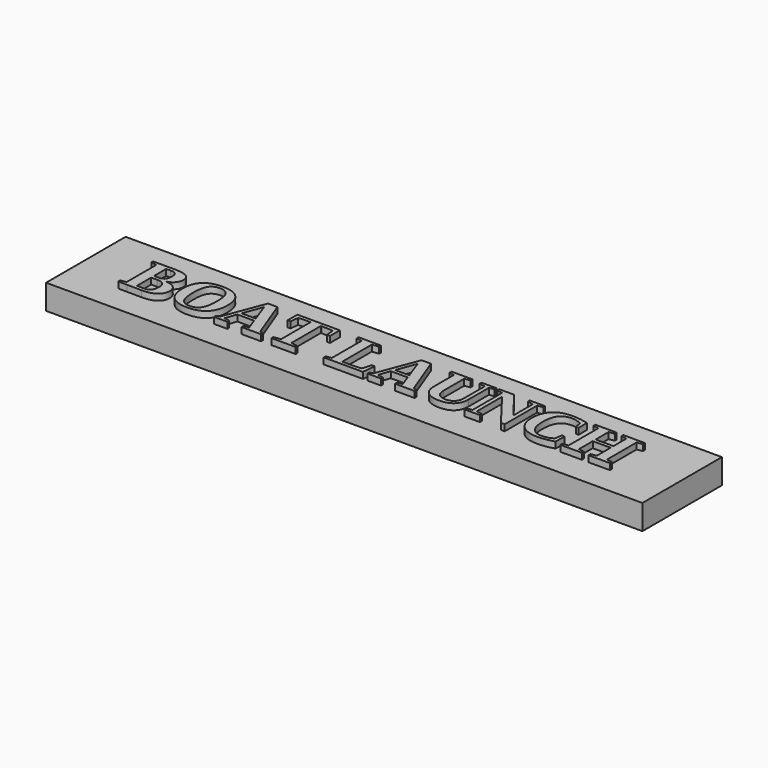
from build123d import *

# Parameters (mm, degrees)
F1_W         = 609.6
F1_H         = 101.6
F2_DEPTH     = 25.4
F0_TEXT_SIZE = 68.0637260033
F3_DEPTH     = 6.35


# Not quite as in the source:
# - Text() gives the source's letters only with a copy of the font that has no kerning and outlines rounded to 1/6400 em; it was checked with that copy


with BuildPart() as f2:
    # F1 (on Top) → F2 (new body)
    with BuildSketch(Plane.XY):
        with Locations((20.5955467701, 29.6312676191)):
            Rectangle(F1_W, F1_H)
    extrude(amount=-F2_DEPTH)

    # F0 (on Top) → F3 (join)
    with BuildSketch(Plane.XY):
        with Locations((-233.9750987422, 6.9081966477)):
            Text('BOAT LAUNCH', F0_TEXT_SIZE, font='Tinos', font_style=FontStyle.BOLD, text_align=(TextAlign.LEFT, TextAlign.BOTTOM))
    extrude(amount=F3_DEPTH)


solid = f2.part
